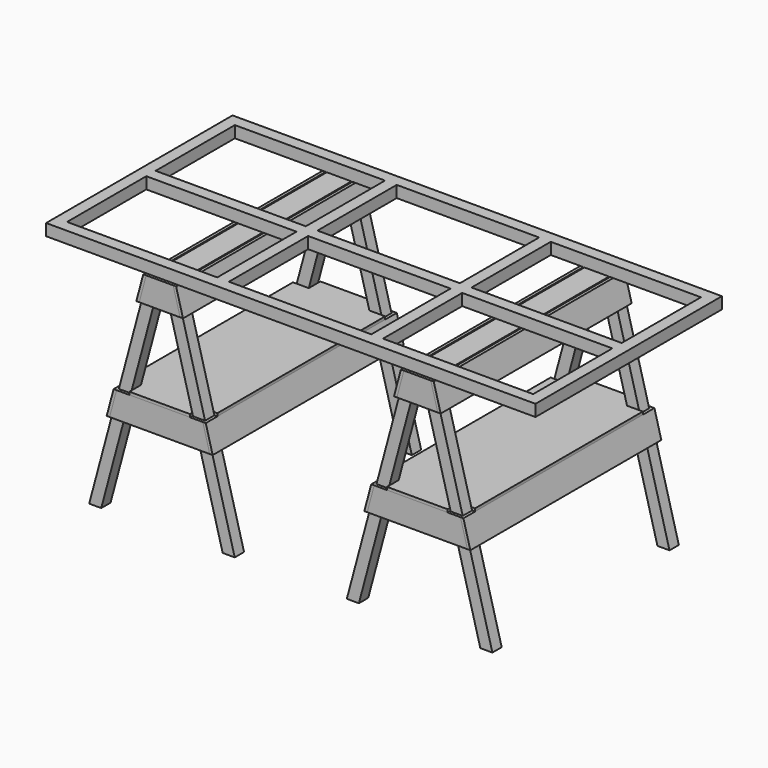
from build123d import *

# Parameters (mm, degrees)
F0_W      = 1890
F0_H      = 900
F0_W_2    = 45
F0_H_2    = 382.5
F0_W_3    = 580
F0_H_3    = 45
F0_W_4    = 550
F1_DEPTH  = 45
F2_W      = 95
F2_H      = 22
F3_DEPTH  = 900
F5_DEPTH  = 45
F7_DEPTH  = 11
F10_DEPTH = 922
F11_W     = 355.8419104132
F11_H     = 922
F12_DEPTH = 11
F14_W     = 80.4998734839
F14_H     = 84.9716675282
F14_W_2   = 86.1553862937
F14_H_2   = 108.1925344467
F14_W_3   = 84.9872687705
F14_H_3   = 77.3259413242
F14_W_4   = 99.3894949801
F14_H_4   = 102.0654153824
F15_DEPTH = 438.501


# Not quite as in the source:
# - a feature names something its author has since deleted; it is built from what else it names


with BuildPart() as f1:
    # F0 (on Top) → F1 (new body)
    with BuildSketch(Plane.XY):
        Rectangle(F0_W, F0_H)
        Polygon((320, 405), (900, 405), (900, 22.5), (900, -22.5), (900, -405), (320, -405), (275, -405), (-275, -405), (-320, -405), (-900, -405), (-900, -22.5), (-900, 22.5), (-900, 405), (-320, 405), (-275, 405), (275, 405), align=None, mode=Mode.SUBTRACT)
        with Locations((297.5, 213.75)):
            Rectangle(F0_W_2, F0_H_2)
        with Locations((610, 0)):
            Rectangle(F0_W_3, F0_H_3)
        with Locations((297.5, 0)):
            Rectangle(F0_W_2, F0_H_3)
        with Locations((-297.5, 213.75)):
            Rectangle(F0_W_2, F0_H_2)
        Rectangle(F0_W_4, F0_H_3)
        with Locations((297.5, -213.75)):
            Rectangle(F0_W_2, F0_H_2)
        with Locations((-297.5, 0)):
            Rectangle(F0_W_2, F0_H_3)
        with Locations((-610, 0)):
            Rectangle(F0_W_3, F0_H_3)
        with Locations((-297.5, -213.75)):
            Rectangle(F0_W_2, F0_H_2)
    extrude(amount=F1_DEPTH)


with BuildPart() as f3:
    # F2 (on face) → F3 (new body, through all)
    with BuildSketch(Plane.XZ.offset(450)):
        with Locations((-497.5, -11)):
            Rectangle(F2_W, F2_H)
    extrude(amount=-F3_DEPTH)


with BuildPart() as f5:
    # F4 (on face) → F5 (new body)
    with BuildSketch(Plane.XZ.offset(450)):
        Polygon((-545, 0), (-549.4846374578, 0), (-778.5811969864, -855), (-731.9937688679, -855), (-508.7920915728, -22), (-545, -22), align=None)
    extrude(amount=-F5_DEPTH)


with BuildPart() as f5b:
    # F4 (on face) → F5, piece 2 (new body)
    with BuildSketch(Plane.XZ.offset(450)):
        Polygon((-450, 0), (-450, -22), (-486.2079084272, -22), (-263.0062311321, -855), (-216.4188030136, -855), (-445.5153625422, 0), align=None)
    extrude(amount=-F5_DEPTH)


with BuildPart() as f7:
    # F6 (on face) → F7 (new body)
    with BuildSketch(Plane.XZ.offset(450)):
        Polygon((-330.9670827779, -427.5), (-664.0329172221, -427.5), (-690.8278364652, -527.5), (-304.1721635348, -527.5), align=None)
    extrude(amount=F7_DEPTH)


with BuildPart() as f7b:
    # F6 (on face) → F7, piece 2 (new body)
    with BuildSketch(Plane.XZ.offset(450)):
        Polygon((-445.5153625422, 0), (-549.4846374578, 0), (-576.2795567009, -100), (-418.7204432991, -100), align=None)
    extrude(amount=F7_DEPTH)


with BuildPart() as f8_1:
    # F8: instance of F5
    add(f5.part.mirror(Plane.XZ))


with BuildPart() as f8_2:
    # F8: instance of F5b
    add(f5b.part.mirror(Plane.XZ))


with BuildPart() as f8_3:
    # F8: instance of F7
    add(f7.part.mirror(Plane.XZ))


with BuildPart() as f8_4:
    # F8: instance of F7b
    add(f7b.part.mirror(Plane.XZ))


with BuildPart() as f10:
    # F9 (on face) → F10 (new body, through all)
    with BuildSketch(Plane(origin=(0, 461, 0), x_dir=(-1, 0, 0), z_dir=(0, 1, 0))):
        Polygon((418.7204432991, -100), (445.5153625422, 0), (434.1273245577, 0), (407.3324053146, -100), align=None)
    extrude(amount=-F10_DEPTH)


with BuildPart() as f10b:
    # F9 (on face) → F10, piece 2 (new body, through all)
    with BuildSketch(Plane(origin=(0, 461, 0), x_dir=(-1, 0, 0), z_dir=(0, 1, 0))):
        Polygon((560.8726754423, 0), (549.4846374578, 0), (576.2795567009, -100), (587.6675946854, -100), align=None)
    extrude(amount=-F10_DEPTH)


with BuildPart() as f10c:
    # F9 (on face) → F10, piece 3 (new body, through all)
    with BuildSketch(Plane(origin=(0, 461, 0), x_dir=(-1, 0, 0), z_dir=(0, 1, 0))):
        Polygon((304.1721635348, -527.5), (330.9670827779, -427.5), (319.5790447934, -427.5), (292.7841255503, -527.5), align=None)
    extrude(amount=-F10_DEPTH)


with BuildPart() as f10d:
    # F9 (on face) → F10, piece 4 (new body, through all)
    with BuildSketch(Plane(origin=(0, 461, 0), x_dir=(-1, 0, 0), z_dir=(0, 1, 0))):
        Polygon((675.4209552066, -427.5), (664.0329172221, -427.5), (690.8278364652, -527.5), (702.2158744497, -527.5), align=None)
    extrude(amount=-F10_DEPTH)


with BuildPart() as f12:
    # F11 (on face) → F12 (new body)
    with BuildSketch(Plane.XY.offset(-427.5)):
        with Locations((-497.5, 0)):
            Rectangle(F11_W, F11_H)
    extrude(amount=F12_DEPTH)

    # F13: cut F5, F5b, F8_1, F8_2
    add(f5.part, mode=Mode.SUBTRACT)
    add(f5b.part, mode=Mode.SUBTRACT)
    add(f8_1.part, mode=Mode.SUBTRACT)
    add(f8_2.part, mode=Mode.SUBTRACT)

    # F14 (on face) → F15 (cut, through all)
    with BuildSketch(Plane.XY.offset(-416.5)):
        with Locations((-654.7479847288, -447.4858337641)):
            Rectangle(F14_W, F14_H)
        with Locations((-337.4242588663, -459.0962672234)):
            Rectangle(F14_W_2, F14_H_2)
        with Locations((-656.9916823721, 443.6629706621)):
            Rectangle(F14_W_3, F14_H_3)
        with Locations((-330.8072045231, 456.0327076912)):
            Rectangle(F14_W_4, F14_H_4)
    extrude(amount=-F15_DEPTH, mode=Mode.SUBTRACT)


with BuildPart() as f16_1:
    # F16: instance of F5b
    add(f5b.part.mirror(Plane.YZ))


with BuildPart() as f16_2:
    # F16: instance of F5
    add(f5.part.mirror(Plane.YZ))


with BuildPart() as f16_3:
    # F16: instance of F3
    add(f3.part.mirror(Plane.YZ))


with BuildPart() as f16_4:
    # F16: instance of F8_3
    add(f8_3.part.mirror(Plane.YZ))


with BuildPart() as f16_5:
    # F16: instance of F8_1
    add(f8_1.part.mirror(Plane.YZ))


with BuildPart() as f16_6:
    # F16: instance of F8_2
    add(f8_2.part.mirror(Plane.YZ))


with BuildPart() as f16_7:
    # F16: instance of F8_4
    add(f8_4.part.mirror(Plane.YZ))


with BuildPart() as f16_8:
    # F16: instance of F7
    add(f7.part.mirror(Plane.YZ))


with BuildPart() as f16_9:
    # F16: instance of F7b
    add(f7b.part.mirror(Plane.YZ))


with BuildPart() as f16_10:
    # F16: instance of F12
    add(f12.part.mirror(Plane.YZ))


with BuildPart() as f16_11:
    # F16: instance of F10d
    add(f10d.part.mirror(Plane.YZ))


with BuildPart() as f16_12:
    # F16: instance of F10c
    add(f10c.part.mirror(Plane.YZ))


with BuildPart() as f16_13:
    # F16: instance of F10b
    add(f10b.part.mirror(Plane.YZ))


with BuildPart() as f16_14:
    # F16: instance of F10
    add(f10.part.mirror(Plane.YZ))


solid = Compound([f1.part, f3.part, f5.part, f5b.part, f7.part, f7b.part, f8_1.part, f8_2.part, f8_3.part, f8_4.part, f10.part, f10b.part, f10c.part, f10d.part, f12.part, f16_1.part, f16_2.part, f16_3.part, f16_4.part, f16_5.part, f16_6.part, f16_7.part, f16_8.part, f16_9.part, f16_10.part, f16_11.part, f16_12.part, f16_13.part, f16_14.part])
